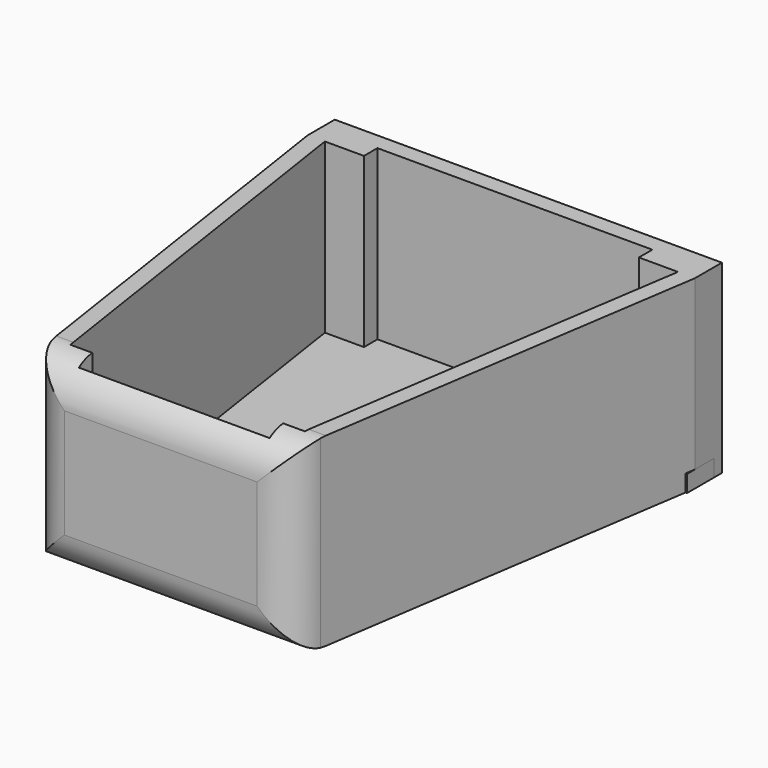
from build123d import *

# Parameters (mm, degrees)
F0_W          = 34
F0_H          = 3
F1_DEPTH      = 33
F3_DEPTH      = 3
F4_T1_DEPTH   = 62.0637231031
F4_T3_DEPTH   = 79.7989898732
F4_2_T1_DEPTH = 62.0886043833


# Not quite as in the source:
# - a fillet or chamfer that OpenCascade refuses, or shapes differently, is made with other operations: its cross-section is extruded or revolved along the edge and cut away or added


with BuildPart() as f1:
    # F0 (on Top) → F1 (new body)
    with BuildSketch(Plane.XY):
        Polygon((-34.5, 39.400604268), (-34.5, 36.400604268), (-24.5, 36.400604268), (24.5, 36.400604268), (34.5, 36.400604268), (34.5, 39.400604268), align=None)
        Polygon((-24.5, 36.400604268), (-34.5, 36.400604268), (-34.5, 33.400604268), (-31.4657606752, 33.400604268), (-24.5, 33.400604268), align=None)
        Polygon((34.5, 36.400604268), (24.5, 36.400604268), (24.5, 33.400604268), (31.4657606752, 33.400604268), (34.5, 33.400604268), align=None)
        Polygon((-23, -39.5), (-23, -42.5), (-17, -42.5), (-17, -39.5), (-20.4203025109, -39.5), align=None)
        Polygon((-17, -36.5), (-20.8748443467, -36.5), (-20.4203025109, -39.5), (-17, -39.5), align=None)
        Polygon((-20.4203025109, -39.5), (-20.8748443467, -36.5), (-23, -36.5), (-23, -39.5), align=None)
        Polygon((20.4203025109, -39.5), (20.8748443467, -36.5), (17, -36.5), (17, -39.5), align=None)
        Polygon((17, -39.5), (17, -42.5), (23, -42.5), (23, -39.5), (20.4203025109, -39.5), align=None)
        Polygon((23, -36.5), (20.8748443467, -36.5), (20.4203025109, -39.5), (23, -39.5), align=None)
        Polygon((23, -42.5), (34.5, 33.400604268), (31.4657606752, 33.400604268), (20.8748443467, -36.5), (23, -36.5), (23, -39.5), align=None)
        Polygon((-31.4657606752, 33.400604268), (-34.5, 33.400604268), (-23, -42.5), (-23, -39.5), (-23, -36.5), (-20.8748443467, -36.5), align=None)
        with Locations((0, -41)):
            Rectangle(F0_W, F0_H)
    extrude(amount=F1_DEPTH)

    # F4: fillet of radius 6.7597979746 on 4 edges, made by hand

    # F4_s2 → F4_t1 (cut)
    with BuildSketch(Plane.XY.offset(-14.5318615516)):
        with BuildLine():
            ThreePointArc((-23.8707736364, -36.7528482447), (-21.5946120019, -40.8656362762), (-17.1872553794, -42.5))
            Line((-17.1872553794, -42.5), (-23, -42.5))
            Line((-23, -42.5), (-23.8707736364, -36.7528482447))
        make_face()
        with BuildLine():
            ThreePointArc((17.1872553794, -42.5), (21.5946120019, -40.8656362762), (23.8707736364, -36.7528482447))
            Line((23.8707736364, -36.7528482447), (23, -42.5))
            Line((23, -42.5), (17.1872553794, -42.5))
        make_face()
    extrude(amount=F4_T1_DEPTH, mode=Mode.SUBTRACT)

    # F4_s4 → F4_t3 (cut)
    with BuildSketch(Plane.YZ.offset(-39.8994949366)):
        with BuildLine():
            ThreePointArc((-42.5, 6.7597979746), (-40.5201010127, 1.9798989873), (-35.7402020254, 0))
            Line((-35.7402020254, 0), (-42.5, 0))
            Line((-42.5, 0), (-42.5, 6.7597979746))
        make_face()
        with BuildLine():
            ThreePointArc((-42.5, 26.2402020254), (-40.5201010127, 31.0201010127), (-35.7402020254, 33))
            Line((-35.7402020254, 33), (-42.5, 33))
            Line((-42.5, 33), (-42.5, 26.2402020254))
        make_face()
    extrude(amount=F4_T3_DEPTH, mode=Mode.SUBTRACT)


with BuildPart() as f3:
    # F2 (on Top) → F3 (new body)
    with BuildSketch(Plane.XY):
        Polygon((24.5, 34.6106770507), (-24.5, 34.6106770507), (-24.5, 31.6106770507), (-31.4657606752, 31.6106770507), (-20.8748443467, -38.2899272173), (-17, -38.2899272173), (-17, -41.2899272173), (17, -41.2899272173), (17, -38.2899272173), (20.8748443467, -38.2899272173), (31.4657606752, 31.6106770507), (24.5, 31.6106770507), align=None)
        Polygon((-34.5, 37.6106770507), (-34.5, 34.6106770507), (-24.5, 34.6106770507), (24.5, 34.6106770507), (34.5, 34.6106770507), (34.5, 37.6106770507), align=None)
        Polygon((34.5, 34.6106770507), (24.5, 34.6106770507), (24.5, 31.6106770507), (31.4657606752, 31.6106770507), (34.5, 31.6106770507), align=None)
        Polygon((-24.5, 34.6106770507), (-34.5, 34.6106770507), (-34.5, 31.6106770507), (-31.4657606752, 31.6106770507), (-24.5, 31.6106770507), align=None)
    extrude(amount=F3_DEPTH)

    # F4#2: fillet of radius 6.7597979746 on 1 edges, made by hand

    # F4_2_s2 → F4_2_t1 (cut)
    with BuildSketch(Plane.YZ.offset(-31.0443021916)):
        with BuildLine():
            ThreePointArc((-41.2899272173, 3), (-38.8564954233, 0.7969822223), (-35.6722063406, 0))
            Line((-35.6722063406, 0), (-41.2899272173, 0))
            Line((-41.2899272173, 0), (-41.2899272173, 3))
        make_face()
    extrude(amount=F4_2_T1_DEPTH, mode=Mode.SUBTRACT)


solid = Compound([f1.part, f3.part])
